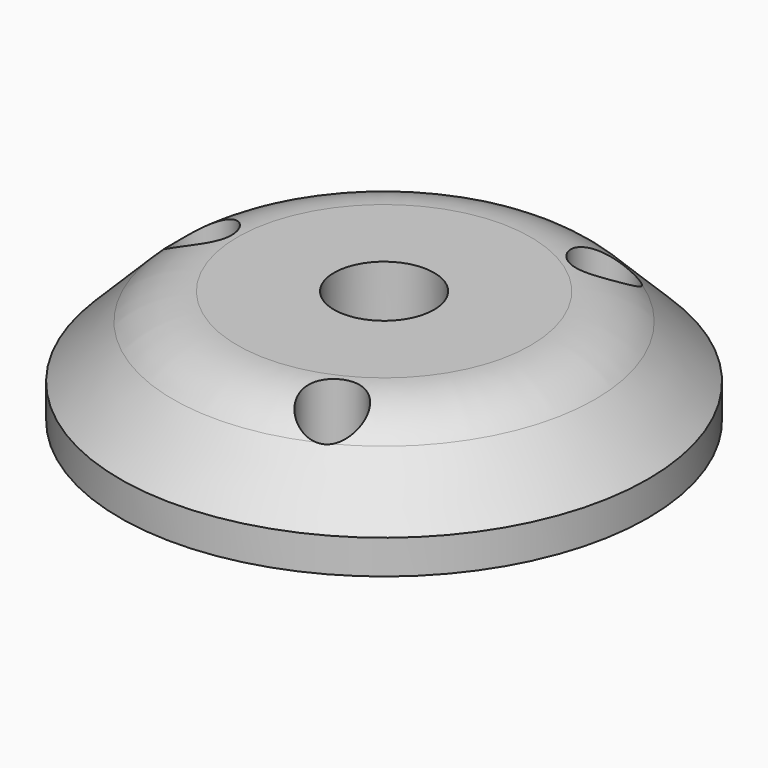
from build123d import *

# Parameters (mm, degrees)
F0_R        = 5.8
F0_R_2      = 1.1
F1_DEPTH    = 2.5
F2_R        = 0.65
F3_DEPTH    = 25
F5_T2_ANGLE = 77.9776147156
F5_T4_ANGLE = 162.2494051266
F5_T6_ANGLE = 155.9758879551
F5_T8_ANGLE = 84.2484124222


# Not quite as in the source:
# - a fillet or chamfer that OpenCascade refuses, or shapes differently, is made with other operations: its cross-section is extruded or revolved along the edge and cut away or added


with BuildPart() as f1:
    # F0 (on Top) → F1 (new body)
    with BuildSketch(Plane.XY):
        Circle(F0_R)
        Circle(F0_R_2, mode=Mode.SUBTRACT)
    extrude(amount=F1_DEPTH)

    # F2 (on face) → F3 (cut)
    with BuildSketch(Plane.XY.offset(2.5)):
        with Locations((-4, 0)):
            Circle(F2_R)
        with Locations((2.125, 3.3888604279)):
            Circle(F2_R)
        with Locations((1.7421875, -3.6006642047)):
            Circle(F2_R)
    extrude(amount=-F3_DEPTH, mode=Mode.SUBTRACT)

    # F4: chamfer of 1.75 on 1 edges, made by hand

    # F4_s1 → F4_t2 (revolve, cut)
    with BuildSketch(Plane.XZ):
        Polygon((5.8, 0.75), (4.05, 2.5), (5.8, 2.5), align=None)
    revolve(axis=Axis((0, 0, 2.5), (0, 0, 1)), mode=Mode.SUBTRACT)

    # F5: fillet of radius 2 on 4 edges, made by hand

    # F5_s1 → F5_t2 (revolve, cut)
    with BuildSketch(Plane.XZ):
        with BuildLine():
            ThreePointArc((4.6357864376, 1.9142135624), (3.98693974, 2.347759065), (3.2215728753, 2.5))
            Line((3.2215728753, 2.5), (4.05, 2.5))
            Line((4.05, 2.5), (4.6357864376, 1.9142135624))
        make_face()
    revolve(axis=Axis((0, 0, 2.5), (0, 0, 1)), revolution_arc=F5_T2_ANGLE, mode=Mode.SUBTRACT)

    # F5_s3 → F5_t4 (revolve, cut)
    with BuildSketch(Plane(origin=(0, 0, 0), x_dir=(0, 0, 1), z_dir=(0.61332513, -0.7898305419, 0))):
        with BuildLine():
            ThreePointArc((1.9142135624, -4.6357864376), (2.347759065, -3.98693974), (2.5, -3.2215728753))
            Line((2.5, -3.2215728753), (2.5, -4.05))
            Line((2.5, -4.05), (1.9142135624, -4.6357864376))
        make_face()
    revolve(axis=Axis((0, 0, 2.5), (0, 0, 1)), revolution_arc=F5_T4_ANGLE, mode=Mode.SUBTRACT)

    # F5_s5 → F5_t6 (revolve, cut)
    with BuildSketch(Plane(origin=(0, 0, 0), x_dir=(0, 0, 1), z_dir=(0.3432973656, 0.9392267664, 0))):
        with BuildLine():
            ThreePointArc((1.9142135624, -4.6357864376), (2.347759065, -3.98693974), (2.5, -3.2215728753))
            Line((2.5, -3.2215728753), (2.5, -4.05))
            Line((2.5, -4.05), (1.9142135624, -4.6357864376))
        make_face()
    revolve(axis=Axis((0, 0, 2.5), (0, 0, 1)), revolution_arc=F5_T6_ANGLE, mode=Mode.SUBTRACT)

    # F5_s7 → F5_t8 (revolve, cut)
    with BuildSketch(Plane(origin=(0, 0, 0), x_dir=(0, 0, 1), z_dir=(-0.9949657418, -0.1002156306, 0))):
        with BuildLine():
            ThreePointArc((1.9142135624, -4.6357864376), (2.347759065, -3.98693974), (2.5, -3.2215728753))
            Line((2.5, -3.2215728753), (2.5, -4.05))
            Line((2.5, -4.05), (1.9142135624, -4.6357864376))
        make_face()
    revolve(axis=Axis((0, 0, 2.5), (0, 0, 1)), revolution_arc=F5_T8_ANGLE, mode=Mode.SUBTRACT)


solid = f1.part
